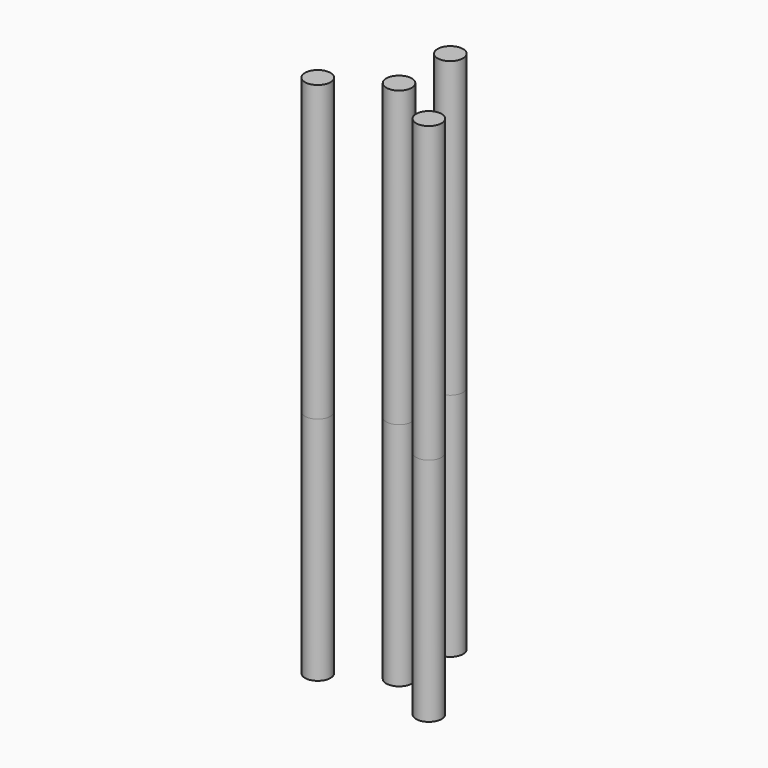
from build123d import *

# Parameters (mm, degrees)
F0_R     = 11.05
F1_DEPTH = 200
F2_DEPTH = 255.3823423


# Not quite as in the source:
# - an extrude ends at something that could not be found from the text; its depth is read off the source's solid


with BuildPart() as f1:
    # F0 (on Top) → F1 (new body)
    with BuildSketch(Plane.XY):
        with Locations((-48.2293143136, -27.8452076018)):
            Circle(F0_R)
    extrude(amount=F1_DEPTH)


with BuildPart() as f1b:
    # F0 (on Top) → F1, piece 2 (new body)
    with BuildSketch(Plane.XY):
        with Locations((-0.1010427902, 0.2113740662)):
            Circle(F0_R)
    extrude(amount=F1_DEPTH)


with BuildPart() as f1c:
    # F0 (on Top) → F1, piece 3 (new body)
    with BuildSketch(Plane.XY):
        with Locations((0, 55.6904152036)):
            Circle(F0_R)
    extrude(amount=F1_DEPTH)


with BuildPart() as f1d:
    # F0 (on Top) → F1, piece 4 (new body)
    with BuildSketch(Plane.XY):
        with Locations((48.2293143136, -27.8452076018)):
            Circle(F0_R)
    extrude(amount=F1_DEPTH)


with BuildPart() as f2:
    # F2 (new, through all): a face of the model
    f2_faces = [f1c.part.faces().sort_by_distance(p)[0] for p in [
        (0, 55.6904152036, 200),
    ]]
    extrude(f2_faces, amount=F2_DEPTH)


with BuildPart() as f2b:
    # F2#2 (new, through all): a face of the model
    f2_2_faces = [f1b.part.faces().sort_by_distance(p)[0] for p in [
        (-0.1010427902, 0.2113740662, 200),
    ]]
    extrude(f2_2_faces, amount=F2_DEPTH)


with BuildPart() as f2c:
    # F2#3 (new, through all): a face of the model
    f2_3_faces = [f1.part.faces().sort_by_distance(p)[0] for p in [
        (-48.2293143136, -27.8452076018, 200),
    ]]
    extrude(f2_3_faces, amount=F2_DEPTH)


with BuildPart() as f2d:
    # F2#4 (new, through all): a face of the model
    f2_4_faces = [f1d.part.faces().sort_by_distance(p)[0] for p in [
        (48.2293143136, -27.8452076018, 200),
    ]]
    extrude(f2_4_faces, amount=F2_DEPTH)


solid = Compound([f1.part, f1b.part, f1c.part, f1d.part, f2.part, f2b.part, f2c.part, f2d.part])
